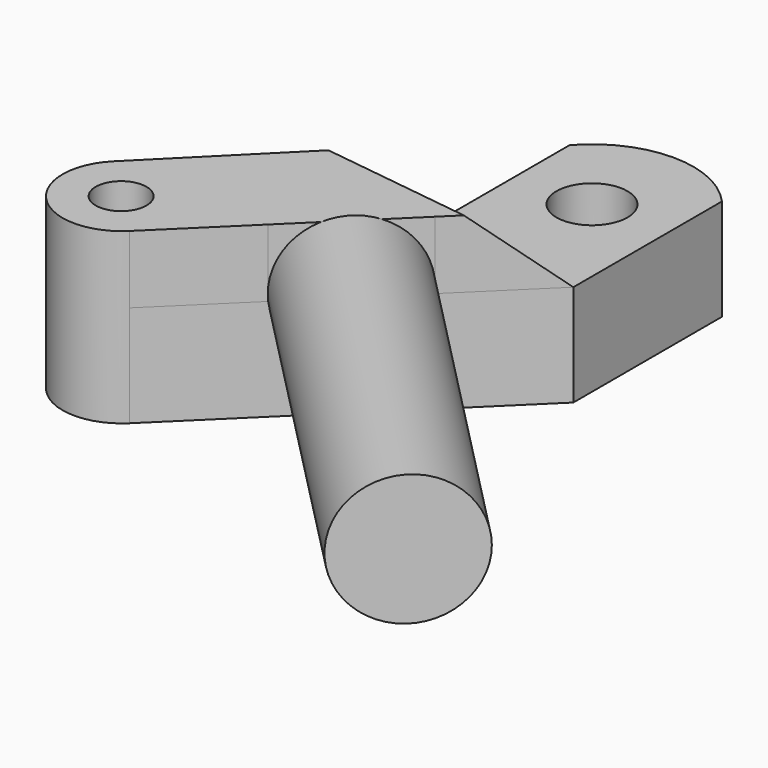
from build123d import *

# Parameters (mm, degrees)
F0_R     = 1.5
F0_R_2   = 2.1
F1_DEPTH = 6
F2_R     = 3.88
F3_DEPTH = 26
F4_R     = 1.5
F5_DEPTH = 4
F6_SIZE  = 3.99999


# Not quite as in the source:
# - a fillet or chamfer is up to 0.001 mm smaller than in the source, because OpenCascade refuses the exact size


with BuildPart() as f1:
    # F0 (on Top) → F1 (new body)
    with BuildSketch(Plane.XY):
        with BuildLine():
            Line((4.5, 0), (4.5, 3.9686269666))
            ThreePointArc((4.5, 3.9686269666), (0, 6), (-4.5, 3.9686269666))
            Line((-4.5, 3.9686269666), (-4.5, 0))
            Line((-4.5, 0), (-4.5, -5.813701588))
            Line((-4.5, -5.813701588), (-15.143203234, -16.4569048219))
            ThreePointArc((-15.143203234, -16.4569048219), (-15.1189316865, -21.3823807428), (-10.1934557657, -21.4066522902))
            Line((-10.1934557657, -21.4066522902), (4.5, -7))
            Line((4.5, -7), (4.5, 0))
        make_face()
        with Locations((-12.6691633098, -18.9323580438)):
            Circle(F0_R, mode=Mode.SUBTRACT)
        Circle(F0_R_2, mode=Mode.SUBTRACT)
    extrude(amount=F1_DEPTH)

    # F2 (on face) → F3 (join)
    with BuildSketch(Plane(origin=(5.7049735344, -5.8185465008, 0), x_dir=(0.7140411723, 0.7001037097, 0), z_dir=(0.7001037097, -0.7140411723, 0))):
        with Locations((-11.9764822387, 6.39)):
            Circle(F2_R)
    extrude(amount=F3_DEPTH)

    # F4 (on face) → F5 (join)
    with BuildSketch(Plane.XY.offset(6)):
        with BuildLine():
            Line((-4.5, -5.813701588), (-15.143203234, -16.4569048219))
            ThreePointArc((-15.143203234, -16.4569048219), (-15.1189316865, -21.3823807428), (-10.1934557657, -21.4066522902))
            Line((-10.1934557657, -21.4066522902), (-5.6031765259, -16.9059713084))
            Line((-5.6031765259, -16.9059713084), (-0.0762481345, -11.4869237515))
            Line((-0.0762481345, -11.4869237515), (4.5, -7))
            Line((4.5, -7), (-4.5, -5.813701588))
        make_face()
        with Locations((-12.6691633098, -18.9323580438)):
            Circle(F4_R, mode=Mode.SUBTRACT)
    extrude(amount=F5_DEPTH)

    # F6 (size 4 in the source; OpenCascade refuses exactly that, so slightly less here)
    f6_edges = [f1.edges().sort_by_distance(p)[0] for p in [
        (0, -6.406851, 10),
    ]]
    chamfer(f6_edges, length=F6_SIZE)


solid = f1.part
